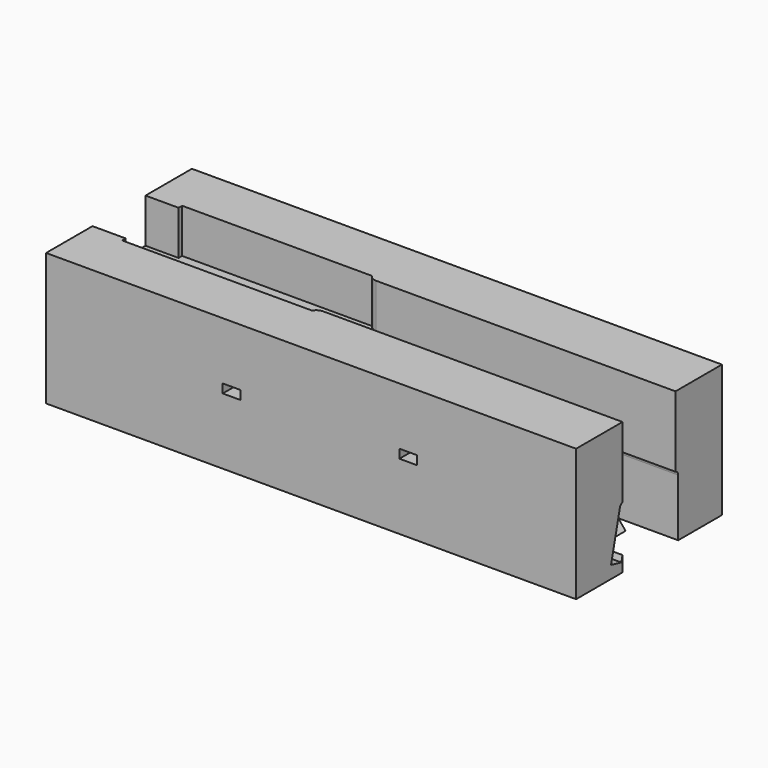
from build123d import *

# Parameters (mm, degrees)
F0_W         = 52.4178380828
F0_H         = 38.1
F1_DEPTH     = 152.4
F3_DEPTH     = 152.401
F5_DEPTH     = 12.7
F7_DEPTH     = 19.05
F8_W         = 5.08
F8_H         = 2.54
F9_DEPTH     = 52.4188380828
F10_R        = 2.54
F11_T1_DEPTH = 18.199261314


# Not quite as in the source:
# - a fillet or chamfer that OpenCascade refuses, or shapes differently, is made with other operations: its cross-section is extruded or revolved along the edge and cut away or added


with BuildPart() as f1:
    # F0 (on Right) → F1 (new body)
    with BuildSketch(Plane.YZ):
        Rectangle(F0_W, F0_H)
    extrude(amount=-F1_DEPTH)

    # F2 (on face) → F3 (cut, through all)
    with BuildSketch(Plane.YZ):
        with BuildLine():
            Line((6.6756140975, -19.05), (10.4856140975, -19.05))
            Line((10.4856140975, -19.05), (10.4856140975, -2.54))
            ThreePointArc((10.4856140975, -2.54), (10.1136397096, -1.6419743879), (9.2156140975, -1.27))
            Line((9.2156140975, -1.27), (-9.2156140975, -1.27))
            ThreePointArc((-9.2156140975, -1.27), (-10.0011773128, -1.5421070023), (-10.4501149349, -2.241826087))
            Line((-10.4501149349, -2.241826087), (-13.6443859025, -15.4667596303))
            Line((-13.6443859025, -15.4667596303), (-9.9408833902, -16.3612813694))
            Line((-9.9408833902, -16.3612813694), (-7.2160704876, -5.08))
            Line((-7.2160704876, -5.08), (6.6756140975, -5.08))
            Line((6.6756140975, -5.08), (6.6756140975, -19.05))
        make_face()
    extrude(amount=-F3_DEPTH, mode=Mode.SUBTRACT)

    # F4 (on face) → F5 (cut)
    with BuildSketch(Plane.XY.offset(19.05)):
        Polygon((-142.875, -10.795), (-88.265, -10.795), (-88.265, -9.525), (0, -9.525), (0, 9.525), (-88.265, 9.525), (-88.265, 10.795), (-142.875, 10.795), (-142.875, 9.525), (-152.4, 9.525), (-152.4, -9.525), (-142.875, -9.525), align=None)
    extrude(amount=-F5_DEPTH, mode=Mode.SUBTRACT)

    # F6 (on face) → F7 (cut, through all)
    with BuildSketch(Plane.XZ.offset(-9.525)):
        Polygon((0, 6.35), (-33.02, 6.35), (-12.065, -19.05), (0, -19.05), align=None)
    extrude(amount=F7_DEPTH, mode=Mode.SUBTRACT)

    # F8 (on face) → F9 (cut, through all)
    with BuildSketch(Plane.XZ.offset(26.2089190414)):
        with Locations((-99.06, 1.27)):
            Rectangle(F8_W, F8_H)
        with Locations((-48.26, 1.27)):
            Rectangle(F8_W, F8_H)
    extrude(amount=-F9_DEPTH, mode=Mode.SUBTRACT)

    # F10
    f10_edges = [f1.edges().sort_by_distance(p)[0] for p in [
        (-87.995125, -7.21607, -5.08),
        (-87.995125, 6.675614, -5.08),
    ]]
    fillet(f10_edges, radius=F10_R)

    # F11: fillet of radius 2.54 on 2 edges, made by hand

    # F11_s2 → F11_t1 (cut)
    with BuildSketch(Plane.XY.offset(6.35)):
        with BuildLine():
            ThreePointArc((-86.0652954744, -9.525), (-87.3352954744, -9.8652954744), (-88.265, -10.795))
            Line((-88.265, -10.795), (-88.265, -9.525))
            Line((-88.265, -9.525), (-86.0652954744, -9.525))
        make_face()
        with BuildLine():
            ThreePointArc((-86.0652954744, 9.525), (-87.3352954744, 9.8652954744), (-88.265, 10.795))
            Line((-88.265, 10.795), (-88.265, 9.525))
            Line((-88.265, 9.525), (-86.0652954744, 9.525))
        make_face()
    extrude(amount=F11_T1_DEPTH, mode=Mode.SUBTRACT)


solid = f1.part
